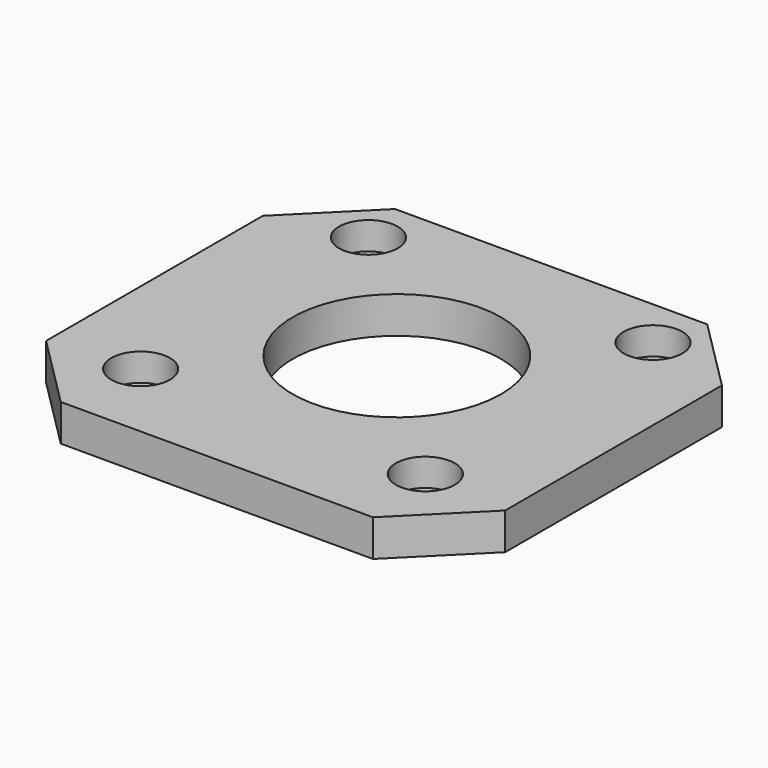
from build123d import *

# Parameters (mm, degrees)
F0_W     = 50
F0_H     = 45.5
F0_R     = 3.2
F0_R_2   = 5
F0_R_3   = 11.35
F1_DEPTH = 4
F0_R_4   = 1.7
F2_DEPTH = 1
F3_DEPTH = 3
F4_SIZE  = 8


# Not quite as in the source:
# - a feature names something its author has since deleted; it is built from what else it names


with BuildPart() as f1:
    # F0 (on Top) → F1 (new body)
    with BuildSketch(Plane.XY):
        with Locations((0, -1.75)):
            Rectangle(F0_W, F0_H)
        with Locations((-15.5, -15.5)):
            Circle(F0_R, mode=Mode.SUBTRACT)
        with Locations((-6.4, -15.4509711824)):
            Circle(F0_R_2, mode=Mode.SUBTRACT)
        with Locations((-15.4509711824, -6.4)):
            Circle(F0_R_2, mode=Mode.SUBTRACT)
        with Locations((6.4, -15.4509711824)):
            Circle(F0_R_2, mode=Mode.SUBTRACT)
        with Locations((15.5, -15.5)):
            Circle(F0_R, mode=Mode.SUBTRACT)
        with Locations((15.4509711824, -6.4)):
            Circle(F0_R_2, mode=Mode.SUBTRACT)
        with Locations((-15.4509711824, 6.4)):
            Circle(F0_R_2, mode=Mode.SUBTRACT)
        with Locations((-15.5, 15.5)):
            Circle(F0_R, mode=Mode.SUBTRACT)
        with Locations((-6.4, 15.4509711824)):
            Circle(F0_R_2, mode=Mode.SUBTRACT)
        Circle(F0_R_3, mode=Mode.SUBTRACT)
        with Locations((15.4509711824, 6.4)):
            Circle(F0_R_2, mode=Mode.SUBTRACT)
        with Locations((6.4, 15.4509711824)):
            Circle(F0_R_2, mode=Mode.SUBTRACT)
        with Locations((15.5, 15.5)):
            Circle(F0_R, mode=Mode.SUBTRACT)
        with Locations((-15.4509711824, -6.4)):
            Circle(F0_R_2)
        with Locations((-6.4, -15.4509711824)):
            Circle(F0_R_2)
        with Locations((6.4, -15.4509711824)):
            Circle(F0_R_2)
        with Locations((15.4509711824, -6.4)):
            Circle(F0_R_2)
        with Locations((15.4509711824, 6.4)):
            Circle(F0_R_2)
        with Locations((6.4, 15.4509711824)):
            Circle(F0_R_2)
        with Locations((-6.4, 15.4509711824)):
            Circle(F0_R_2)
        with Locations((-15.4509711824, 6.4)):
            Circle(F0_R_2)
    extrude(amount=F1_DEPTH)

    # F0 (on Top) → F2 (join)
    with BuildSketch(Plane.XY):
        with Locations((-15.5, 15.5)):
            Circle(F0_R)
        with Locations((-15.5, 15.5)):
            Circle(F0_R_4, mode=Mode.SUBTRACT)
        with Locations((15.5, 15.5)):
            Circle(F0_R)
        with Locations((15.5, 15.5)):
            Circle(F0_R_4, mode=Mode.SUBTRACT)
        with Locations((15.5, -15.5)):
            Circle(F0_R)
        with Locations((15.5, -15.5)):
            Circle(F0_R_4, mode=Mode.SUBTRACT)
        with Locations((-15.5, -15.5)):
            Circle(F0_R)
        with Locations((-15.5, -15.5)):
            Circle(F0_R_4, mode=Mode.SUBTRACT)
    extrude(amount=F2_DEPTH)

    # F0 (on Top) → F3 (cut)
    with BuildSketch(Plane.XY):
        with Locations((-15.4509711824, -6.4)):
            Circle(F0_R_2)
        with Locations((-6.4, -15.4509711824)):
            Circle(F0_R_2)
        with Locations((6.4, -15.4509711824)):
            Circle(F0_R_2)
        with Locations((15.4509711824, -6.4)):
            Circle(F0_R_2)
        with Locations((15.4509711824, 6.4)):
            Circle(F0_R_2)
        with Locations((6.4, 15.4509711824)):
            Circle(F0_R_2)
        with Locations((-6.4, 15.4509711824)):
            Circle(F0_R_2)
        with Locations((-15.4509711824, 6.4)):
            Circle(F0_R_2)
    extrude(amount=F3_DEPTH, mode=Mode.SUBTRACT)

    # F4
    f4_edges = [f1.edges().sort_by_distance(p)[0] for p in [
        (25, 21, 2),
        (-25, 21, 2),
        (25, -24.5, 2),
        (-25, -24.5, 2),
    ]]
    chamfer(f4_edges, length=F4_SIZE)


solid = f1.part
